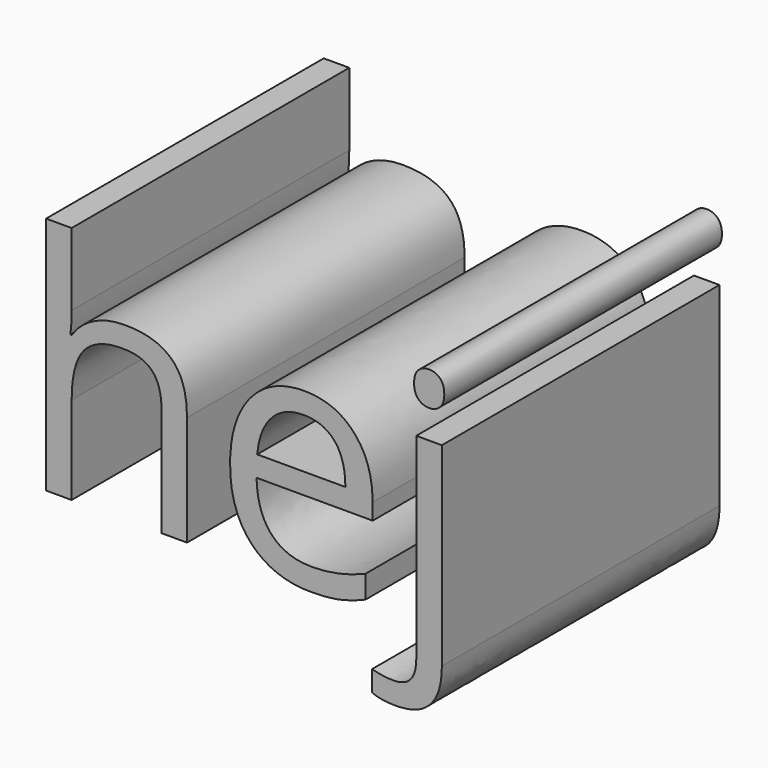
from build123d import *

# Parameters (mm, degrees)
F0_TEXT_SIZE = 23.0602557874
F1_DEPTH     = 25.4


# Not quite as in the source:
# - Text() gives the source's letters only with a copy of the font that has no kerning and outlines rounded to 1/6400 em; it was checked with that copy


with BuildPart() as f1:
    # F0 (on Front) → F1 (new body)
    with BuildSketch(Plane.XZ):
        with Locations((-32.6194524443, -49.9859265983)):
            Text('hej', F0_TEXT_SIZE, font='Open Sans', text_align=(TextAlign.LEFT, TextAlign.BOTTOM))
    extrude(amount=F1_DEPTH)


solid = f1.part
